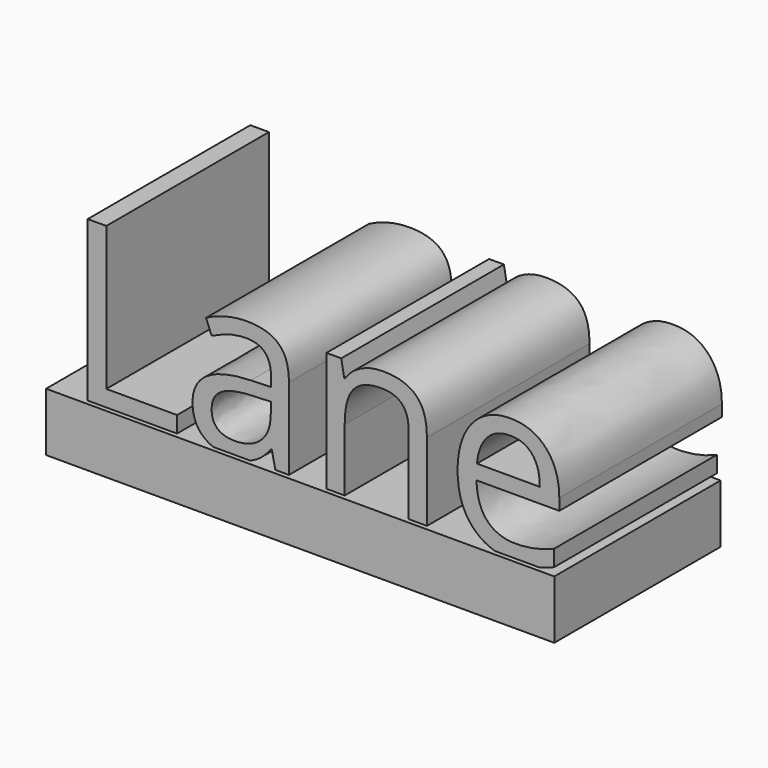
from build123d import *

# Parameters (mm, degrees)
F0_W         = 50.8
F0_H         = 20.780704887
F1_DEPTH     = 5.842
F2_TEXT_SIZE = 22.453038674
F3_DEPTH     = 20.32


# Not quite as in the source:
# - Text() gives the source's letters only with a copy of the font that has no kerning and outlines rounded to 1/6400 em; it was checked with that copy


with BuildPart() as f1:
    # F0 (on Top) → F1 (new body)
    with BuildSketch(Plane.XY):
        with Locations((-1.5868046448, -10.3903524435)):
            Rectangle(F0_W, F0_H)
    extrude(amount=F1_DEPTH)

    # F2 (on Front) → F3 (join)
    with BuildSketch(Plane.XZ):
        with Locations((-25.4, 5.7868587114)):
            Text('Lane', F2_TEXT_SIZE, font='Open Sans', text_align=(TextAlign.LEFT, TextAlign.BOTTOM))
    extrude(amount=F3_DEPTH)


solid = f1.part
